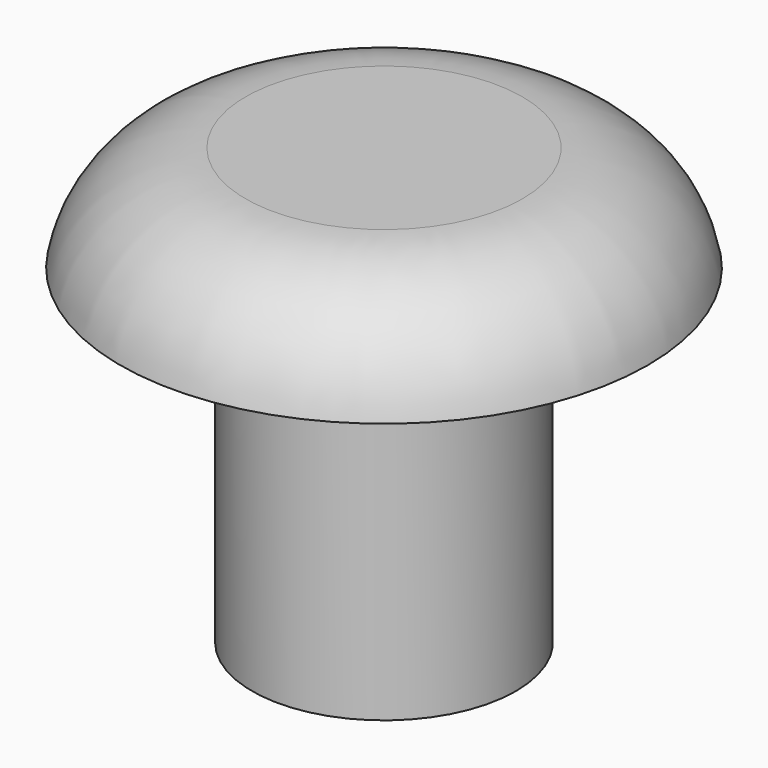
from build123d import *

# Parameters (mm, degrees)
F0_R     = 6.35
F1_DEPTH = 2.54
F3_R     = 3.175
F4_DEPTH = 7.9375


# Not quite as in the source:
# - a fillet or chamfer that OpenCascade refuses, or shapes differently, is made with other operations: its cross-section is extruded or revolved along the edge and cut away or added


with BuildPart() as f1:
    # F0 (on Top) → F1 (new body)
    with BuildSketch(Plane.XY):
        Circle(F0_R)
    extrude(amount=F1_DEPTH)

    # F2: fillet of radius 3.0660512242 on 1 edges, made by hand

    # F2_s1 → F2_t2 (revolve, cut)
    with BuildSketch(Plane.XZ):
        with BuildLine():
            ThreePointArc((6.35, 0), (5.3027068749, 1.8206027884), (3.3294139279, 2.54))
            Line((3.3294139279, 2.54), (6.35, 2.54))
            Line((6.35, 2.54), (6.35, 0))
        make_face()
    revolve(axis=Axis((0, 0, 2.54), (0, 0, 1)), mode=Mode.SUBTRACT)

    # F3 (on face) → F4 (join)
    with BuildSketch(Plane(origin=(0, 0, 0), x_dir=(1, 0, 0), z_dir=(0, 0, -1))):
        Circle(F3_R)
    extrude(amount=F4_DEPTH)


solid = f1.part
